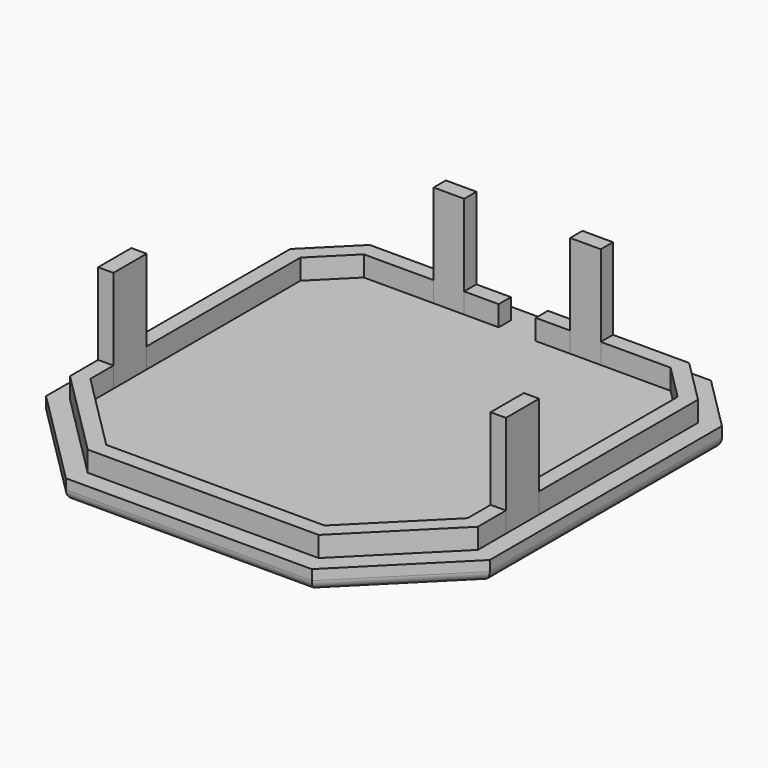
from build123d import *

# Parameters (mm, degrees)
F0_W     = 1.4999995628
F0_H     = 4.0733087808
F0_W_2   = 3
F0_H_2   = 1.4999995628
F0_W_3   = 3.3865806442
F0_W_4   = 3.6284167378
F1_DEPTH = 2
F2_DEPTH = 2
F3_DEPTH = 10
F4_R     = 1


# Not quite as in the source:
# - a feature names something its author has since deleted; it is built from what else it names


with BuildPart() as f1:
    # F0 (on Top) → F1 (new body)
    with BuildSketch(Plane.XY):
        Polygon((-22.7132121537, 14.7005723555), (-22.7132121537, -13.7593665438), (-13.0109889089, -23.4615897885), (11.1091688922, -23.4615897885), (20.811392137, -13.7593665438), (20.811392137, 14.7005723555), (15.4489499903, 20.0630145022), (-17.350770007, 20.0630145022), align=None)
        Polygon((19.0490899916, -13.0293970941), (10.3791994426, -21.6992876432), (-12.2810194593, -21.6992876432), (-20.9509100084, -13.0293970941), (-20.9509100084, -9.5797898248), (-20.9509100084, -5.506481044), (-20.9509100084, 13.9706029059), (-16.6208005574, 18.3007123568), (-9.1516990215, 18.3007123568), (-6.1516990215, 18.3007123568), (-2.7651183773, 18.3007123568), (0.8632983606, 18.3007123568), (4.2498790047, 18.3007123568), (7.2498790047, 18.3007123568), (14.7189805407, 18.3007123568), (19.0490899916, 13.9706029059), (19.0490899916, -5.506481044), (19.0490899916, -9.5797898248), align=None, mode=Mode.SUBTRACT)
        Polygon((-12.2810194593, -21.6992876432), (10.3791994426, -21.6992876432), (19.0490899916, -13.0293970941), (19.0490899916, -9.5797898248), (17.5490904289, -9.5797898248), (17.5490904289, -12.4080769317), (9.7578792802, -20.1992880804), (-11.6596992969, -20.1992880804), (-19.4509104456, -12.4080769317), (-19.4509104456, -9.5797898248), (-20.9509100084, -9.5797898248), (-20.9509100084, -13.0293970941), align=None)
        with Locations((18.2990902103, -7.5431354344)):
            Rectangle(F0_W, F0_H)
        Polygon((17.5490904289, -5.506481044), (19.0490899916, -5.506481044), (19.0490899916, 13.9706029059), (14.7189805407, 18.3007123568), (7.2498790047, 18.3007123568), (7.2498790047, 16.8007127941), (14.0976603782, 16.8007127941), (17.5490904289, 13.3492827434), align=None)
        Polygon((17.5490904289, -12.4080769317), (17.5490904289, -9.5797898248), (17.5490904289, -5.506481044), (17.5490904289, 13.3492827434), (14.0976603782, 16.8007127941), (7.2498790047, 16.8007127941), (4.2498790047, 16.8007127941), (0.8632983606, 16.8007127941), (-2.7651183773, 16.8007127941), (-6.1516990215, 16.8007127941), (-9.1516990215, 16.8007127941), (-15.9994803949, 16.8007127941), (-19.4509104456, 13.3492827434), (-19.4509104456, -5.506481044), (-19.4509104456, -9.5797898248), (-19.4509104456, -12.4080769317), (-11.6596992969, -20.1992880804), (9.7578792802, -20.1992880804), align=None)
        Polygon((-20.9509100084, 13.9706029059), (-20.9509100084, -5.506481044), (-19.4509104456, -5.506481044), (-19.4509104456, 13.3492827434), (-15.9994803949, 16.8007127941), (-9.1516990215, 16.8007127941), (-9.1516990215, 18.3007123568), (-16.6208005574, 18.3007123568), align=None)
        with Locations((-20.200910227, -7.5431354344)):
            Rectangle(F0_W, F0_H)
        with Locations((5.7498790047, 17.5507125754)):
            Rectangle(F0_W_2, F0_H_2)
        with Locations((-4.4584086994, 17.5507125754)):
            Rectangle(F0_W_3, F0_H_2)
        with Locations((-7.6516990215, 17.5507125754)):
            Rectangle(F0_W_2, F0_H_2)
        with Locations((2.5565886827, 17.5507125754)):
            Rectangle(F0_W_3, F0_H_2)
        with Locations((-0.9509100084, 17.5507125754)):
            Rectangle(F0_W_4, F0_H_2)
    extrude(amount=-F1_DEPTH)

    # F0 (on Top) → F2 (join)
    with BuildSketch(Plane.XY):
        Polygon((-12.2810194593, -21.6992876432), (10.3791994426, -21.6992876432), (19.0490899916, -13.0293970941), (19.0490899916, -9.5797898248), (17.5490904289, -9.5797898248), (17.5490904289, -12.4080769317), (9.7578792802, -20.1992880804), (-11.6596992969, -20.1992880804), (-19.4509104456, -12.4080769317), (-19.4509104456, -9.5797898248), (-20.9509100084, -9.5797898248), (-20.9509100084, -13.0293970941), align=None)
        Polygon((-20.9509100084, 13.9706029059), (-20.9509100084, -5.506481044), (-19.4509104456, -5.506481044), (-19.4509104456, 13.3492827434), (-15.9994803949, 16.8007127941), (-9.1516990215, 16.8007127941), (-9.1516990215, 18.3007123568), (-16.6208005574, 18.3007123568), align=None)
        Polygon((17.5490904289, -5.506481044), (19.0490899916, -5.506481044), (19.0490899916, 13.9706029059), (14.7189805407, 18.3007123568), (7.2498790047, 18.3007123568), (7.2498790047, 16.8007127941), (14.0976603782, 16.8007127941), (17.5490904289, 13.3492827434), align=None)
        with Locations((-4.4584086994, 17.5507125754)):
            Rectangle(F0_W_3, F0_H_2)
        with Locations((2.5565886827, 17.5507125754)):
            Rectangle(F0_W_3, F0_H_2)
    extrude(amount=F2_DEPTH)

    # F4
    f4_edges = [f1.edges().sort_by_distance(p)[0] for p in [
        (-22.713212, 0.470603, -2),
        (-17.862101, -18.610478, -2),
        (-0.95091, -23.46159, -2),
        (15.960281, -18.610478, -2),
        (20.811392, 0.470603, -2),
        (18.130171, 17.381793, -2),
        (-0.95091, 20.063015, -2),
        (-20.031991, 17.381793, -2),
    ]]
    fillet(f4_edges, radius=F4_R)


with BuildPart() as f3:
    # F0 (on Top) → F3 (new body)
    with BuildSketch(Plane.XY):
        with Locations((-20.200910227, -7.5431354344)):
            Rectangle(F0_W, F0_H)
    extrude(amount=F3_DEPTH)


with BuildPart() as f3b:
    # F0 (on Top) → F3, piece 2 (new body)
    with BuildSketch(Plane.XY):
        with Locations((18.2990902103, -7.5431354344)):
            Rectangle(F0_W, F0_H)
    extrude(amount=F3_DEPTH)


with BuildPart() as f3c:
    # F0 (on Top) → F3, piece 3 (new body)
    with BuildSketch(Plane.XY):
        with Locations((-7.6516990215, 17.5507125754)):
            Rectangle(F0_W_2, F0_H_2)
    extrude(amount=F3_DEPTH)


with BuildPart() as f3d:
    # F0 (on Top) → F3, piece 4 (new body)
    with BuildSketch(Plane.XY):
        with Locations((5.7498790047, 17.5507125754)):
            Rectangle(F0_W_2, F0_H_2)
    extrude(amount=F3_DEPTH)


solid = Compound([f1.part, f3.part, f3b.part, f3c.part, f3d.part])
